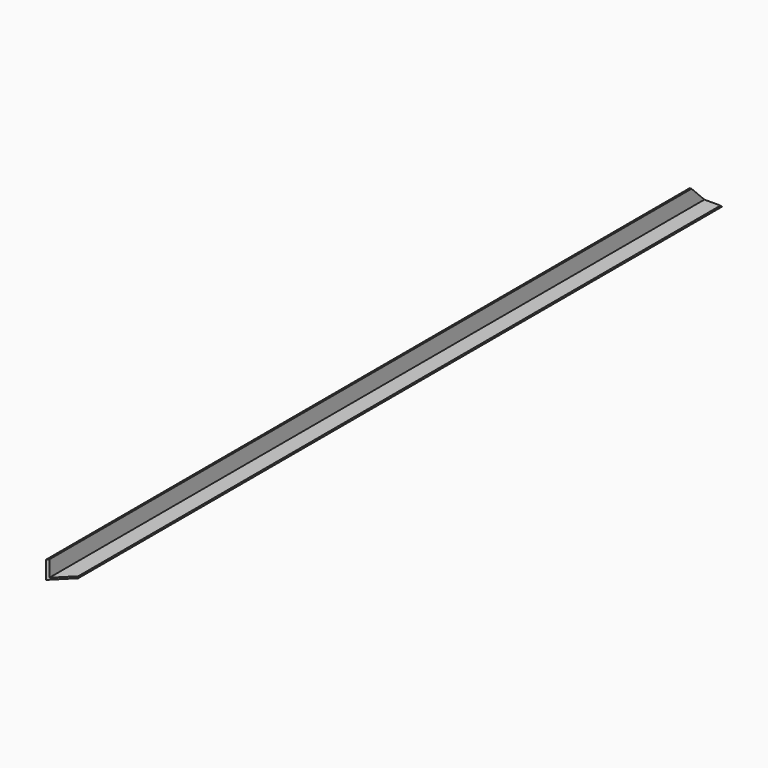
from build123d import *

# Parameters (mm, degrees)
F1_DEPTH = 1380
F2_SIZE  = 29.99999
F3_SIZE  = 29.99999


# Not quite as in the source:
# - a fillet or chamfer is up to 0.001 mm smaller than in the source, because OpenCascade refuses the exact size


with BuildPart() as f1:
    # F0 (on Front) → F1 (new body)
    with BuildSketch(Plane.XZ):
        Polygon((-30, 0), (0, 0), (0, 3), (-27, 3), (-27, 30), (-30, 30), align=None)
    extrude(amount=-F1_DEPTH)

    # F2 (size 30 in the source; OpenCascade refuses exactly that, so slightly less here)
    f2_edges = [f1.edges().sort_by_distance(p)[0] for p in [
        (0, 0, 1.5),
    ]]
    chamfer(f2_edges, length=F2_SIZE)

    # F3 (size 30 in the source; OpenCascade refuses exactly that, so slightly less here)
    f3_edges = [f1.edges().sort_by_distance(p)[0] for p in [
        (-28.5, 1380, 30),
    ]]
    chamfer(f3_edges, length=F3_SIZE)


solid = f1.part
